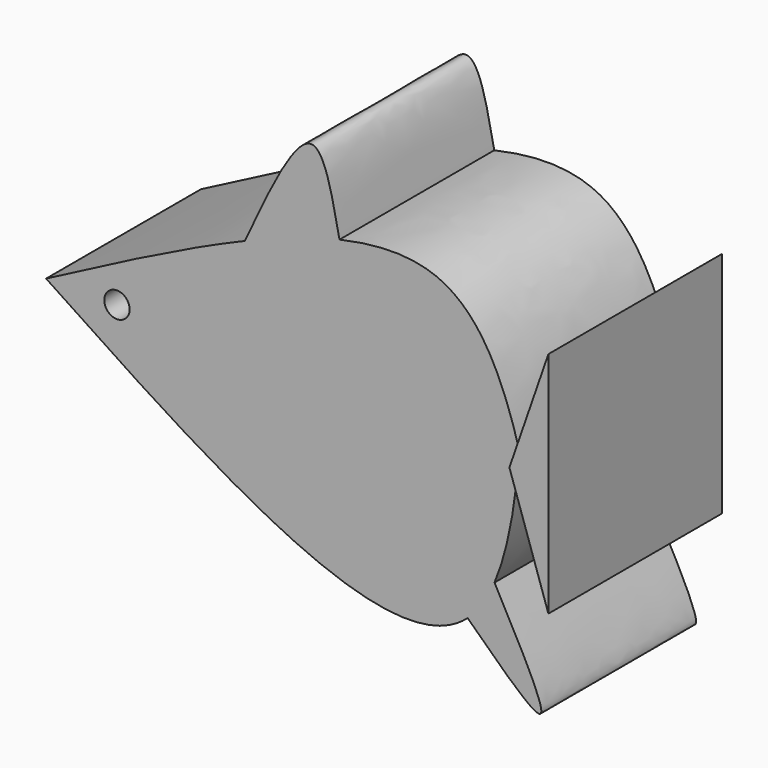
from build123d import *

# Parameters (mm, degrees)
F1_DEPTH = 48.26
F2_R     = 3.163158907
F3_DEPTH = 219.202
F7_DEPTH = 54.102


# Not quite as in the source:
# - the program builds the solid bodies; features that only make, move or delete a surface that nothing else refers to are left out


with BuildPart() as f1:
    # F0 (on Front) → F1 (new body)
    with BuildSketch(Plane.XZ):
        with BuildLine():
            add(Edge.make_bspline(
                [(-55.6729212403, 0), (-38.6311113221, 8.9523120314), (-21.5893014039, 17.9046240629), (-6.1160224097, 24.3814345232)],
                knots=[0, 0, 0, 0, 0.2526308872, 0.2526308872, 0.2526308872, 0.2526308872], degree=3))
            add(Edge.make_bspline(
                [(-55.6729212403, 0), (-31.4820105475, -16.1714644762), (-7.2910998546, -32.3429289523), (12.6646309673, -40.3317198143)],
                knots=[0, 0, 0, 0, 0.2592898959, 0.2592898959, 0.2592898959, 0.2592898959], degree=3))
            add(Edge.make_bspline(
                [(12.6646309673, -40.3317198143), (12.7977790108, -40.2702503671), (12.8467772947, -40.3473806791), (12.8960343857, -40.4240649186)],
                knots=[0.9475980683, 0.9475980683, 0.9475980683, 0.9475980683, 1, 1, 1, 1], degree=3))
            add(Edge.make_bspline(
                [(12.8960343857, -40.4240649186), (28.2628150861, -46.5369934422), (41.10024341, -47.763030362), (49.4649163881, -40.3473806791)],
                knots=[0.2602929484, 0.2602929484, 0.2602929484, 0.2602929484, 0.4602864698, 0.4602864698, 0.4602864698, 0.4602864698], degree=3))
            add(Edge.make_bspline(
                [(49.4649163881, -40.3473806791), (50.5850376596, -39.3543440149), (53.1057014839, -36.5716905465), (55.1277076242, -32.8255943911), (56.1638529866, -30.3775797313)],
                knots=[0.4602864698, 0.4602864698, 0.4602864698, 0.4602864698, 0.4870677915, 0.5252020603, 0.5252020603, 0.5252020603, 0.5252020603], degree=3))
            add(Edge.make_bspline(
                [(56.1638529866, -30.3775797313), (59.780967595, -21.8317232251), (61.5497398481, -10.2709798617), (62.3385554338, 0.6850550301)],
                knots=[0.5252020603, 0.5252020603, 0.5252020603, 0.5252020603, 0.658326259, 0.658326259, 0.658326259, 0.658326259], degree=3))
            add(Edge.make_bspline(
                [(17.5085796013, 32.359251714), (27.1297909673, 34.5637852704), (49.1028218124, 35.1002074944), (58.1974759597, 15.3115973831), (62.3385554338, 0.6850550301)],
                knots=[0.3901714972, 0.3901714972, 0.3901714972, 0.3901714972, 0.5729185448, 0.8708638911, 0.8708638911, 0.8708638911, 0.8708638911], degree=3))
            add(Edge.make_bspline(
                [(-6.1160224097, 24.3814345232), (2.3081424102, 27.9076243402), (10.2673831039, 30.7000572468), (17.5085796013, 32.359251714)],
                knots=[0.2526308872, 0.2526308872, 0.2526308872, 0.2526308872, 0.3901714972, 0.3901714972, 0.3901714972, 0.3901714972], degree=3))
        make_face()
        with BuildLine():
            add(Edge.make_bspline(
                [(-6.1160224097, 24.3814345232), (0.1635435456, 37.996667677), (11.5728562583, 62.1838548689), (15.6705155598, 41.5433244951), (17.5085796013, 32.359251714)],
                knots=[0, 0, 0, 0, 0.556951444, 1, 1, 1, 1], degree=3))
            add(Edge.make_bspline(
                [(-6.1160224097, 24.3814345232), (2.3081424102, 27.9076243402), (10.2673831039, 30.7000572468), (17.5085796013, 32.359251714)],
                knots=[0.2526308872, 0.2526308872, 0.2526308872, 0.2526308872, 0.3901714972, 0.3901714972, 0.3901714972, 0.3901714972], degree=3))
        make_face()
        with BuildLine():
            add(Edge.make_bspline(
                [(49.4649163881, -40.3473806791), (50.5850376596, -39.3543440149), (53.1057014839, -36.5716905465), (55.1277076242, -32.8255943911), (56.1638529866, -30.3775797313)],
                knots=[0.4602864698, 0.4602864698, 0.4602864698, 0.4602864698, 0.4870677915, 0.5252020603, 0.5252020603, 0.5252020603, 0.5252020603], degree=3))
            add(Edge.make_bspline(
                [(49.4649163881, -40.3473806791), (57.8118629624, -48.4510792467), (75.1782729057, -65.3113945884), (62.6635379474, -42.3189795748), (56.1638529866, -30.3775797313)],
                knots=[0, 0, 0, 0, 0.480637426, 1, 1, 1, 1], degree=3))
        make_face()
    extrude(amount=F1_DEPTH)

    # F2 (on Front) → F3 (cut)
    with BuildSketch(Plane.XZ):
        with Locations((-37.9989780486, 0)):
            Circle(F2_R)
    extrude(amount=F3_DEPTH, mode=Mode.SUBTRACT)


with BuildPart() as f7:
    # F4 (on Front) → F7 (new body)
    with BuildSketch(Plane.XZ):
        Polygon((74.2782354355, 28.057385236), (64.5575672388, 0), (74.2782354355, -28.9410892874), align=None)
    extrude(amount=F7_DEPTH)


solid = Compound([f1.part, f7.part])
